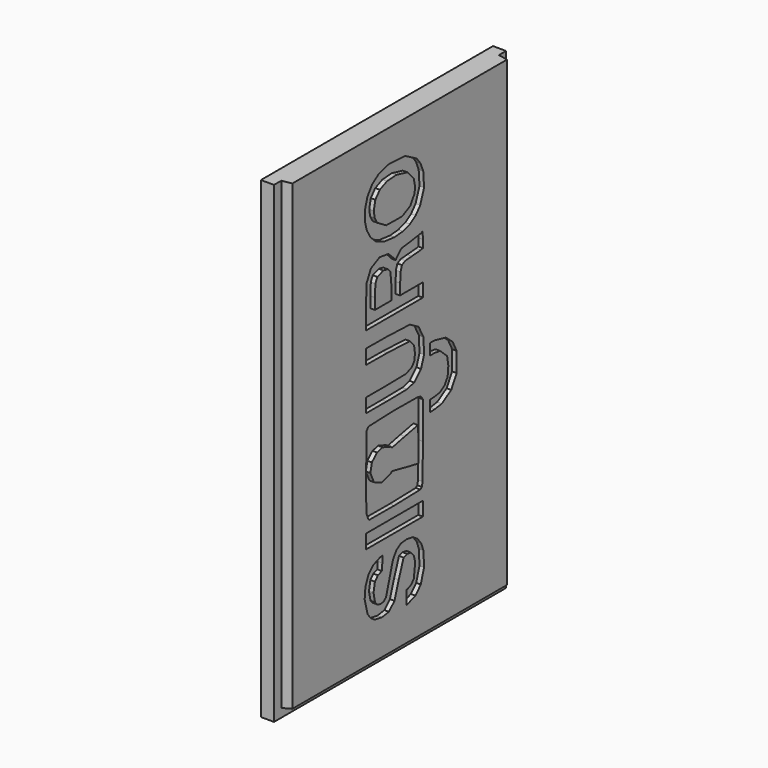
from build123d import *

# Parameters (mm, degrees)
F0_W         = 1.7
F0_H         = 47.6
F1_DEPTH     = 82.8
F2_DEPTH     = 1.5
F3_T4_DEPTH  = 90.1422275002
F3_T9_DEPTH  = 56.4422275002
F3_T14_DEPTH = 90.1422275002
F5_DEPTH     = 0.8


# Not quite as in the source:
# - a fillet or chamfer that OpenCascade refuses, or shapes differently, is made with other operations: its cross-section is extruded or revolved along the edge and cut away or added
# - ends of sketch curves that miss each other by under 0.0002 mm in the source are joined


with BuildPart() as f1:
    # F0 (on Top) → F1 (new body)
    with BuildSketch(Plane.XY):
        Polygon((21.457163617, -2.1686828911), (21.457163617, -52.9686828911), (23.757163617, -52.9686828911), (23.757163617, -51.3686828911), (23.757163617, -3.7686828911), (23.757163617, -2.1686828911), align=None)
        with Locations((24.607163617, -27.5686828911)):
            Rectangle(F0_W, F0_H)
    extrude(amount=F1_DEPTH)

    # F0 (on Top) → F2 (cut)
    with BuildSketch(Plane.XY):
        with Locations((24.607163617, -27.5686828911)):
            Rectangle(F0_W, F0_H)
    extrude(amount=F2_DEPTH, mode=Mode.SUBTRACT)

    # F3: chamfer of 0.3 x 1.7013845459 on 3 edges, made by hand


with BuildPart() as f3_tool2:
    # F3_s3 → F3_t4 (new body)
    with BuildSketch(Plane.XY.offset(-2.9211137501)):
        Polygon((25.457163617, -51.0686828911), (23.7557790711, -51.3686828911), (25.457163617, -51.3686828911), align=None)
    extrude(amount=F3_T4_DEPTH)

    split(bisect_by=Plane.YZ.offset(23.757163617), keep=Keep.TOP)


with BuildPart() as f1_1:
    add(f1.part)

    # F3_t1: cut F3_tool2
    add(f3_tool2.part, mode=Mode.SUBTRACT)


with BuildPart() as f3_tool7:
    # F3_s8 → F3_t9 (new body)
    with BuildSketch(Plane.XZ.offset(55.7897966412)):
        Polygon((23.7557790711, 1.5), (25.457163617, 1.8), (25.457163617, 1.5), align=None)
    extrude(amount=-F3_T9_DEPTH)

    split(bisect_by=Plane.YZ.offset(23.757163617), keep=Keep.TOP)


with BuildPart() as f1_2:
    add(f1_1.part)

    # F3_t6: cut F3_tool7
    add(f3_tool7.part, mode=Mode.SUBTRACT)


with BuildPart() as f3_tool12:
    # F3_s13 → F3_t14 (new body)
    with BuildSketch(Plane.XY.offset(-2.9211137501)):
        Polygon((23.7557790711, -3.7686828911), (25.457163617, -4.0686828911), (25.457163617, -3.7686828911), align=None)
    extrude(amount=F3_T14_DEPTH)

    split(bisect_by=Plane.YZ.offset(23.757163617), keep=Keep.TOP)


with BuildPart() as f1_3:
    add(f1_2.part)

    # F3_t11: cut F3_tool12
    add(f3_tool12.part, mode=Mode.SUBTRACT)

    # F4 (on face) → F5 (cut)
    with BuildSketch(Plane.YZ.offset(25.457163617)):
        Polygon((-22.505932635, 22.2772588), (-28.724640035, 22.2772588), (-34.943347435, 22.2772588), (-34.943347435, 21.0504388), (-34.943347435, 19.8236188), (-28.724640035, 19.8236188), (-22.505932635, 19.8236188), (-22.505932635, 21.0504388), align=None)
        Polygon((-22.252491435, 11.9033908), (-22.383707835, 14.55891), (-22.877052035, 15.8481378), (-23.652310835, 16.8536222), (-24.679334435, 17.5437148), (-26.017177835, 17.7722386), (-27.310164835, 17.6454926), (-28.280495635, 17.045824), (-29.052122235, 15.8700834), (-29.831368835, 13.1980288), (-30.578357435, 10.6597814), (-31.121434835, 10.2112174), (-31.809419235, 10.1062392), (-32.482214435, 10.3308006), (-32.979800435, 10.87083), (-33.312388035, 12.4693028), (-33.006114835, 14.0530944), (-32.346019635, 14.7798392), (-31.495551435, 15.085071), (-31.389811235, 16.2572556), (-31.389811235, 17.4289576), (-31.861946435, 17.354942), (-33.325011835, 16.7950498), (-34.421174235, 15.690607), (-35.085155635, 14.1400894), (-35.251652635, 12.2419982), (-34.630673435, 9.7362374), (-33.962958235, 8.840227), (-33.012566435, 8.2039062), (-31.432102235, 7.9361394), (-29.937820235, 8.1714196), (-28.720017235, 9.3681914), (-27.795787435, 12.2355466), (-26.728733435, 15.2197418), (-25.952255435, 15.4869498), (-25.086471035, 15.3216466), (-24.499985035, 14.6215718), (-24.182434235, 13.5052164), (-24.496632235, 11.0541418), (-25.052739835, 10.3807116), (-25.825687235, 10.038345), (-26.144076235, 9.987418), (-26.144076235, 8.815843), (-26.144076235, 7.6442426), (-25.869121235, 7.6895816), (-24.128662435, 8.3000706), (-22.969762035, 9.542791), align=None)
        Polygon((-22.505881835, 37.9047866), (-22.697931235, 38.1922638), (-22.988278635, 38.5414122), (-23.676618635, 38.7122018), (-28.824233435, 38.7556104), (-34.408398035, 38.558354), (-34.795163835, 38.0930006), (-34.943220435, 31.4334), (-34.890769435, 25.4484234), (-34.482134235, 24.3078618), (-34.252924635, 24.0963306), (-28.794236035, 24.073369), (-23.057976235, 24.221959), (-22.730494035, 24.4872874), (-22.568746835, 25.2639432), (-22.507863035, 31.4235956), align=None)
        Polygon((-23.436614035, 31.4199634), (-23.501028435, 28.4238556), (-25.497722435, 28.7969054), (-28.339398235, 29.390986), (-29.248769035, 29.5721642), (-29.638125635, 29.2749588), (-31.506473435, 28.7259886), (-33.215283835, 29.4793526), (-33.990441035, 31.1879344), (-33.676598635, 32.7156174), (-32.537357835, 33.7839922), (-31.313712835, 34.0783782), (-29.541605635, 33.456002), (-29.229820635, 33.2090632), (-26.481286635, 33.7904438), (-23.584670635, 34.3740342), align=None, mode=Mode.SUBTRACT)
        Polygon((-15.109681235, 38.9450944), (-15.105083835, 42.3673126), (-15.995480835, 44.1325618), (-17.479526635, 45.3944338), (-19.985465235, 45.9675848), (-20.898366635, 45.9675848), (-20.898366635, 44.9946124), (-20.898366635, 44.0216146), (-20.055467635, 44.0216146), (-18.748129635, 43.8478278), (-17.201015635, 42.4311936), (-16.935712635, 40.8064826), (-17.087045835, 39.1853022), (-17.764032035, 38.1211946), (-18.794992635, 37.4568576), (-20.031134435, 37.2759588), (-20.898366635, 37.2286386), (-20.898366635, 36.2548788), (-20.898366635, 35.281119), (-19.904210635, 35.331792), (-18.360119235, 35.5539912), (-16.300890435, 36.8370976), align=None)
        Polygon((-22.252389835, 44.687374), (-22.382818835, 47.453688), (-23.444183235, 49.469813), (-25.347202035, 50.5905626), (-30.395655235, 50.7693786), (-34.943347435, 50.804202), (-34.943347435, 49.5308746), (-34.943347435, 48.2575472), (-30.311047835, 48.2336204), (-25.340293235, 48.0275756), (-24.436840635, 47.0241486), (-24.242327435, 45.713788), (-24.380605035, 44.5729978), (-24.959928235, 43.8294128), (-26.208414435, 43.3369576), (-30.612723635, 43.2601226), (-34.943347435, 43.2601226), (-34.943347435, 42.0333026), (-34.943347435, 40.8064826), (-30.480262635, 40.807905), (-25.970924435, 40.8769676), (-24.414742635, 41.2803958), (-22.908675035, 42.7524274), align=None)
        Polygon((-22.505932635, 55.951385), (-25.011058435, 55.951385), (-27.516184235, 55.951385), (-27.477373035, 57.833906), (-27.397998035, 59.5566102), (-27.099954435, 60.4642284), (-26.355759835, 60.8358812), (-24.937982635, 60.9507654), (-22.970828835, 61.1125888), (-22.505932635, 61.2090834), (-22.505932635, 62.5568328), (-22.569381835, 63.903109), (-22.827750635, 63.6960736), (-25.086471035, 63.3630034), (-27.192842235, 63.0905122), (-28.157762835, 62.2060842), (-28.479123635, 61.7905656), (-28.727205435, 62.1334656), (-30.044474835, 63.3909688), (-31.987727235, 63.663333), (-33.890873035, 62.703721), (-34.864404235, 60.7441872), (-34.943347435, 56.9551422), (-34.943347435, 53.5823524), (-28.724640035, 53.5823524), (-22.505932635, 53.5823524), (-22.505932635, 54.766856), align=None)
        Polygon((-29.346000235, 55.951385), (-31.171676035, 55.951385), (-32.997351835, 55.951385), (-32.997351835, 57.8397226), (-32.904692635, 59.978428), (-32.470886035, 60.8346366), (-31.148384235, 61.281702), (-30.191718635, 61.0931832), (-29.615316435, 60.4805098), (-29.373737035, 58.0057116), align=None, mode=Mode.SUBTRACT)
        Polygon((-22.249824435, 70.4248892), (-22.427446635, 73.0456104), (-22.994450835, 74.4503574), (-23.844461835, 75.5792604), (-26.406966235, 77.0228948), (-30.194080835, 77.1960212), (-32.111552235, 76.624191), (-33.600576435, 75.5856104), (-34.639157035, 74.1022758), (-35.205246835, 72.1961836), (-35.214492435, 70.5444978), (-34.785384835, 68.9424944), (-33.978604635, 67.5379252), (-32.854883235, 66.4784912), (-31.035354235, 65.6822012), (-28.713616435, 65.4275154), (-26.863531235, 65.5841064), (-25.333892435, 66.0648522), (-24.089597235, 66.8862374), (-23.095517435, 68.064772), align=None)
        Polygon((-24.229703635, 71.534031), (-24.308926235, 70.4194028), (-25.277885435, 68.8458728), (-27.074783035, 67.954536), (-30.538631835, 67.9974366), (-32.552521635, 69.2239264), (-33.073958235, 70.1835384), (-33.251174035, 71.3487126), (-32.909163035, 72.909441), (-31.930221635, 74.0513996), (-30.384911035, 74.7238646), (-28.343894035, 74.8760614), (-25.904249435, 74.2938172), (-24.520101835, 72.8221666), align=None, mode=Mode.SUBTRACT)
    extrude(amount=-F5_DEPTH, mode=Mode.SUBTRACT)


solid = f1_3.part
